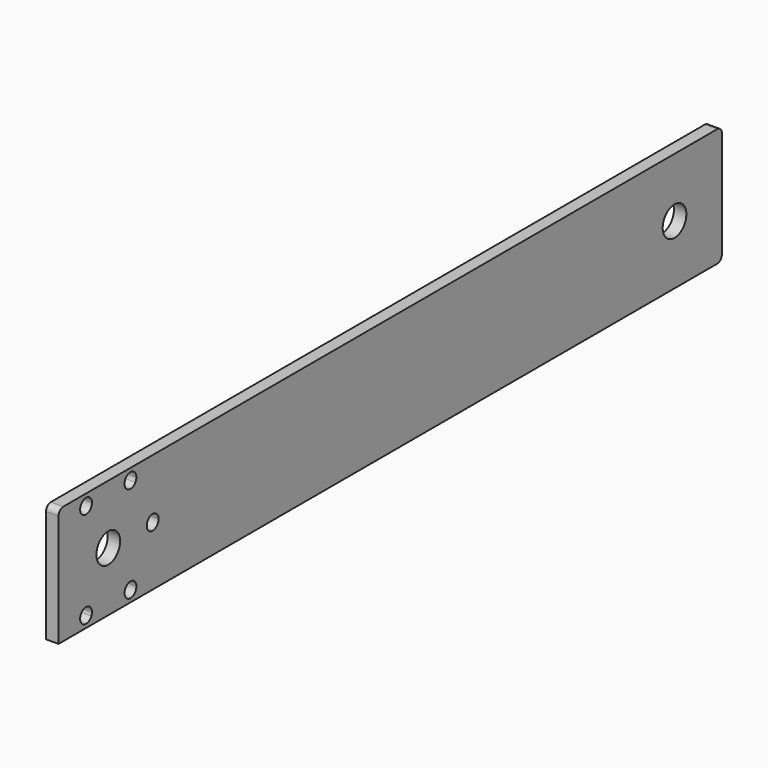
from build123d import *

# Parameters (mm, degrees)
F0_W     = 355.6
F0_H     = 50.8
F0_R     = 6.35
F1_DEPTH = 5.334
F2_R     = 2.54
F4_DEPTH = 25.4


with BuildPart() as f1:
    # F0 (on Right) → F1 (new body)
    with BuildSketch(Plane.YZ):
        with Locations((-62.0332211256, -100.6222862377)):
            Rectangle(F0_W, F0_H)
        with Locations((-213.1684422493, -100.6222862377)):
            Circle(F0_R, mode=Mode.SUBTRACT)
        with Locations((90.3667788744, -100.6222862377)):
            Circle(F0_R, mode=Mode.SUBTRACT)
    extrude(amount=F1_DEPTH)

    # F2
    f2_edges = [f1.edges().sort_by_distance(p)[0] for p in [
        (2.667, 115.766779, -126.022286),
        (2.667, 115.766779, -75.222286),
        (2.667, -239.833221, -75.222286),
    ]]
    fillet(f2_edges, radius=F2_R)

    # F3 (on face) → F4 (cut)
    with BuildSketch(Plane.YZ.offset(5.334)):
        with BuildLine():
            ThreePointArc((-204.111539145, -78.5993967268), (-201.2621922493, -80.0000563101), (-198.6245120203, -81.7673333143))
            ThreePointArc((-198.6245120203, -81.7673333143), (-198.2244908381, -80.9236336682), (-198.0871922493, -80.0000563101))
            ThreePointArc((-198.0871922493, -80.0000563101), (-200.5431829982, -76.9075410398), (-204.111539145, -78.5993967268))
        make_face()
        with BuildLine():
            ThreePointArc((-227.7123724783, -81.7673333143), (-225.0746922493, -80.0000563101), (-222.2253453536, -78.5993967268))
            ThreePointArc((-222.2253453536, -78.5993967268), (-226.6621922493, -77.2504256531), (-227.7123724783, -81.7673333143))
        make_face()
        with BuildLine():
            ThreePointArc((-221.8996922493, -80.0000563101), (-221.982176979, -79.281047059), (-222.2253453536, -78.5993967268))
            ThreePointArc((-222.2253453536, -78.5993967268), (-225.0746922493, -80.0000563101), (-227.7123724783, -81.7673333143))
            ThreePointArc((-227.7123724783, -81.7673333143), (-224.1511148912, -83.0377577213), (-221.8996922493, -80.0000563101))
        make_face()
        with BuildLine():
            ThreePointArc((-204.111539145, -78.5993967268), (-202.8496922493, -82.7496869671), (-198.6245120203, -81.7673333143))
            ThreePointArc((-198.6245120203, -81.7673333143), (-201.2621922493, -80.0000563101), (-204.111539145, -78.5993967268))
        make_face()
        with BuildLine():
            ThreePointArc((-189.567608916, -103.7902228252), (-189.4089178433, -102.2097862377), (-189.3559422493, -100.6222862377))
            ThreePointArc((-189.3559422493, -100.6222862377), (-189.4089178433, -99.0347862377), (-189.567608916, -97.4543496502))
            ThreePointArc((-189.567608916, -97.4543496502), (-192.5309422493, -100.6222862377), (-189.567608916, -103.7902228252))
        make_face()
        with BuildLine():
            ThreePointArc((-189.567608916, -97.4543496502), (-189.4089178433, -99.0347862377), (-189.3559422493, -100.6222862377))
            ThreePointArc((-189.3559422493, -100.6222862377), (-189.4089178433, -102.2097862377), (-189.567608916, -103.7902228252))
            ThreePointArc((-189.567608916, -103.7902228252), (-187.1870043372, -102.9409783978), (-186.1809422493, -100.6222862377))
            ThreePointArc((-186.1809422493, -100.6222862377), (-187.1870043372, -98.3035940776), (-189.567608916, -97.4543496502))
        make_face()
        with BuildLine():
            ThreePointArc((-198.0871922493, -121.2445161653), (-198.2244908381, -120.3209388072), (-198.6245120203, -119.4772391611))
            ThreePointArc((-198.6245120203, -119.4772391611), (-201.2621922493, -121.2445161653), (-204.111539145, -122.6451757486))
            ThreePointArc((-204.111539145, -122.6451757486), (-200.5431829982, -124.3370314356), (-198.0871922493, -121.2445161653))
        make_face()
        with BuildLine():
            ThreePointArc((-204.111539145, -122.6451757486), (-201.2621922493, -121.2445161653), (-198.6245120203, -119.4772391611))
            ThreePointArc((-198.6245120203, -119.4772391611), (-202.8496922493, -118.4948855083), (-204.111539145, -122.6451757486))
        make_face()
        with BuildLine():
            ThreePointArc((-227.7123724783, -119.4772391611), (-226.6621922493, -123.9941468223), (-222.2253453536, -122.6451757486))
            ThreePointArc((-222.2253453536, -122.6451757486), (-225.0746922493, -121.2445161653), (-227.7123724783, -119.4772391611))
        make_face()
        with BuildLine():
            ThreePointArc((-227.7123724783, -119.4772391611), (-225.0746922493, -121.2445161653), (-222.2253453536, -122.6451757486))
            ThreePointArc((-222.2253453536, -122.6451757486), (-221.982176979, -121.9635254164), (-221.8996922493, -121.2445161653))
            ThreePointArc((-221.8996922493, -121.2445161653), (-224.1511148912, -118.2068147541), (-227.7123724783, -119.4772391611))
        make_face()
    extrude(amount=-F4_DEPTH, mode=Mode.SUBTRACT)


solid = f1.part
